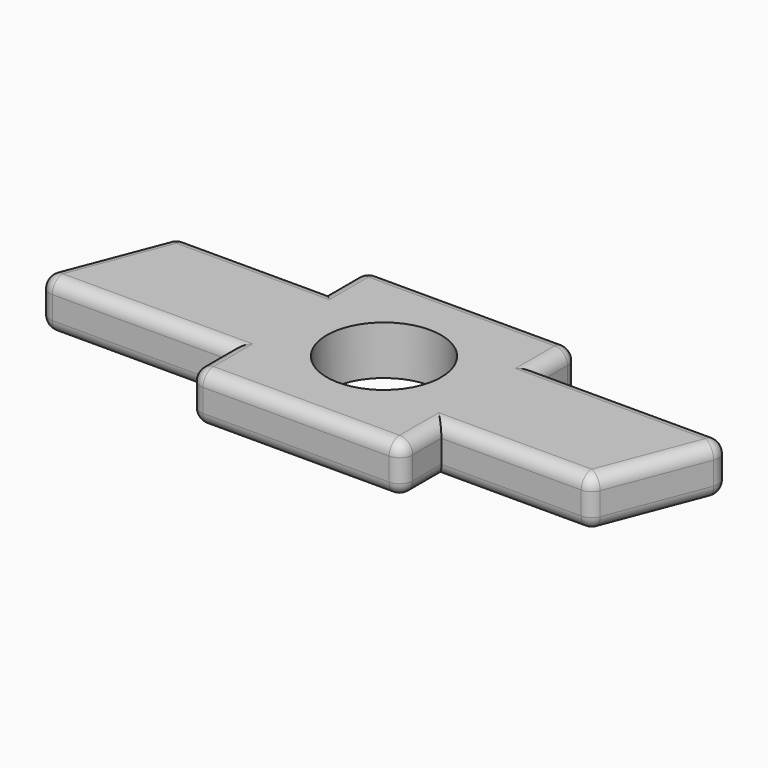
from build123d import *

# Parameters (mm, degrees)
F0_R         = 22.225
F1_DEPTH     = 19.05
F2_R         = 5.08
F3_T1_DEPTH  = 8.89
F3_S5_W      = 5.08
F3_S5_H      = 5.08
F3_T6_DEPTH  = 5.08
F3_S11_W     = 5.08
F3_S11_H     = 5.08
F3_T12_DEPTH = 5.08


# Not quite as in the source:
# - a fillet or chamfer that OpenCascade refuses, or shapes differently, is made with other operations: its cross-section is extruded or revolved along the edge and cut away or added


with BuildPart() as f1:
    # F0 (on Top) → F1 (new body)
    with BuildSketch(Plane.XY):
        Polygon((82.55, 0), (0, 0), (0, -19.05), (-57.8740507578, -19.05), (-76.2, -66.4293159973), (0, -66.4293159973), (0, -85.4793159973), (82.55, -85.4793159973), (82.55, -66.4293159973), (140.4240507578, -66.4293159973), (158.75, -19.05), (82.55, -19.05), align=None)
        with Locations((41.275, -42.7396579986)):
            Circle(F0_R, mode=Mode.SUBTRACT)
    extrude(amount=F1_DEPTH)

    # F2
    f2_edges = [f1.edges().sort_by_distance(p)[0] for p in [
        (111.487025, -66.429316, 19.05),
        (149.587025, -42.739658, 19.05),
        (120.65, -19.05, 19.05),
        (149.587025, -42.739658, 0),
        (111.487025, -66.429316, 0),
        (158.75, -19.05, 9.525),
        (140.424051, -66.429316, 9.525),
        (82.55, -75.954316, 19.05),
        (82.55, -85.479316, 9.525),
        (82.55, -75.954316, 0),
        (41.275, -85.479316, 0),
        (41.275, -85.479316, 19.05),
        (0, -75.954316, 19.05),
        (0, -75.954316, 0),
        (-38.1, -66.429316, 19.05),
        (-76.2, -66.429316, 9.525),
        (-38.1, -66.429316, 0),
        (-67.037025, -42.739658, 19.05),
        (-67.037025, -42.739658, 0),
        (-57.874051, -19.05, 9.525),
        (-28.937025, -19.05, 0),
        (-28.937025, -19.05, 19.05),
        (0, -9.525, 19.05),
        (0, 0, 9.525),
        (0, -9.525, 0),
        (41.275, 0, 19.05),
        (41.275, 0, 0),
        (82.55, -9.525, 19.05),
        (82.55, -9.525, 0),
        (120.65, -19.05, 0),
        (82.55, 0, 9.525),
    ]]
    fillet(f2_edges, radius=F2_R)

    # F3: fillet of radius 5.08 on 1 edges, made by hand

    # F3_s2 → F3_t1 (cut)
    with BuildSketch(Plane.XY.offset(5.08)):
        with BuildLine():
            ThreePointArc((5.08, -85.4793159973), (1.4878975516, -83.9914184457), (0, -80.3993159973))
            Line((0, -80.3993159973), (0, -85.4793159973))
            Line((0, -85.4793159973), (5.08, -85.4793159973))
        make_face()
    extrude(amount=F3_T1_DEPTH, mode=Mode.SUBTRACT)


with BuildPart() as f3_tool4:
    # F3_s5 → F3_t6 (new body)
    with BuildSketch(Plane.XZ.offset(80.3993159973)):
        with Locations((2.54, 2.54)):
            Rectangle(F3_S5_W, F3_S5_H)
    extrude(amount=F3_T6_DEPTH)

    # F3_s7 → F3_t8 (revolve, cut)
    with BuildSketch(Plane(origin=(5.08, -80.3993159973, 5.08), x_dir=(0.7071067812, 0, 0.7071067812), z_dir=(0.7071067812, 0, -0.7071067812))):
        with BuildLine():
            ThreePointArc((0, -5.08), (5.08, 0), (0, 5.08))
            Line((0, 5.08), (0, -5.08))
        make_face()
    revolve(axis=Axis((5.08, -80.3993159973, 5.08), (0, -1, 0)), mode=Mode.SUBTRACT)


with BuildPart() as f1_1:
    add(f1.part)

    # F3_t3: cut F3_tool4
    add(f3_tool4.part, mode=Mode.SUBTRACT)


with BuildPart() as f3_tool10:
    # F3_s11 → F3_t12 (new body)
    with BuildSketch(Plane.XZ.offset(80.3993159973)):
        with Locations((2.54, 16.51)):
            Rectangle(F3_S11_W, F3_S11_H)
    extrude(amount=F3_T12_DEPTH)

    # F3_s13 → F3_t14 (revolve, cut)
    with BuildSketch(Plane(origin=(5.08, -80.3993159973, 13.97), x_dir=(0.7071067812, 0, -0.7071067812), z_dir=(-0.7071067812, 0, -0.7071067812))):
        with BuildLine():
            ThreePointArc((0, -5.08), (5.08, 0), (0, 5.08))
            Line((0, 5.08), (0, -5.08))
        make_face()
    revolve(axis=Axis((5.08, -80.3993159973, 13.97), (0, -1, 0)), mode=Mode.SUBTRACT)


with BuildPart() as f1_2:
    add(f1_1.part)

    # F3_t9: cut F3_tool10
    add(f3_tool10.part, mode=Mode.SUBTRACT)


solid = f1_2.part
